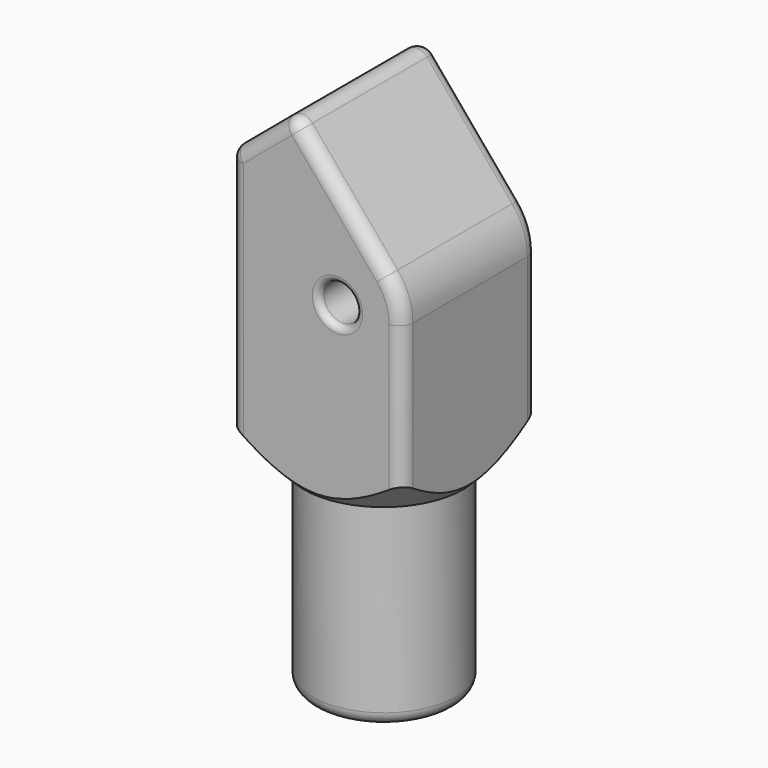
from build123d import *

# Parameters (mm, degrees)
F0_R      = 1.4
F1_DEPTH  = 12.8
F2_R      = 4.9
F3_R      = 1
F4_R      = 5.4
F5_DEPTH  = 15
F9_R      = 3.4
F10_DEPTH = 24
F11_R     = 0.99999
F12_R     = 0.5


# Not quite as in the source:
# - a fillet or chamfer is up to 0.001 mm smaller than in the source, because OpenCascade refuses the exact size


with BuildPart() as f1:
    # F0 (on Front) → F1 (new body)
    with BuildSketch(Plane.XZ):
        Polygon((-13, 0), (0, 0), (0, 15.2073059861), (-8.2170459353, 25), (-13, 20.9866250083), align=None)
        with Locations((-4.9, 13.4238518382)):
            Circle(F0_R, mode=Mode.SUBTRACT)
    extrude(amount=F1_DEPTH)

    # F2
    f2_edges = [f1.edges().sort_by_distance(p)[0] for p in [
        (0, -6.4, 15.207306),
    ]]
    fillet(f2_edges, radius=F2_R)

    # F3
    f3_edges = [f1.edges().sort_by_distance(p)[0] for p in [
        (-8.217046, -6.4, 25),
        (-13, -6.4, 20.986625),
    ]]
    fillet(f3_edges, radius=F3_R)

    # F4 (on face) → F5 (join)
    with BuildSketch(Plane(origin=(0, 0, 0), x_dir=(1, 0, 0), z_dir=(0, 0, -1))):
        with Locations((-6.5, 6.4)):
            Circle(F4_R)
    extrude(amount=F5_DEPTH)

    # F7 (on offset) → F8 (revolve, cut)
    with BuildSketch(Plane.YZ.offset(-6.5)):
        Polygon((-17.45, 0), (-12.45, 0), (-17.45, 5), align=None)
    revolve(axis=Axis((-6.5, -6.45, -7.3510144139), (0, 0, 1)), mode=Mode.SUBTRACT)

    # F9 (on face) → F10 (cut)
    with BuildSketch(Plane(origin=(0, 0, -15), x_dir=(1, 0, 0), z_dir=(0, 0, -1))):
        with Locations((-6.5, 6.4)):
            Circle(F9_R)
    extrude(amount=-F10_DEPTH, mode=Mode.SUBTRACT)

    # F11 (radius 1 in the source; OpenCascade refuses exactly that, so slightly less here)
    f11_edges = [f1.edges().sort_by_distance(p)[0] for p in [
        (-11.9, -6.4, -15),
        (-9.9, -6.4, -15),
        (-13, 0, 11.838709),
        (0, -12.8, 8.255397),
        (-9.9, -6.4, 9),
    ]]
    fillet(f11_edges, radius=F11_R)

    # F12
    f12_edges = [f1.edges().sort_by_distance(p)[0] for p in [
        (-6.3, -12.8, 13.423852),
        (-6.3, 0, 13.423852),
    ]]
    fillet(f12_edges, radius=F12_R)


solid = f1.part
